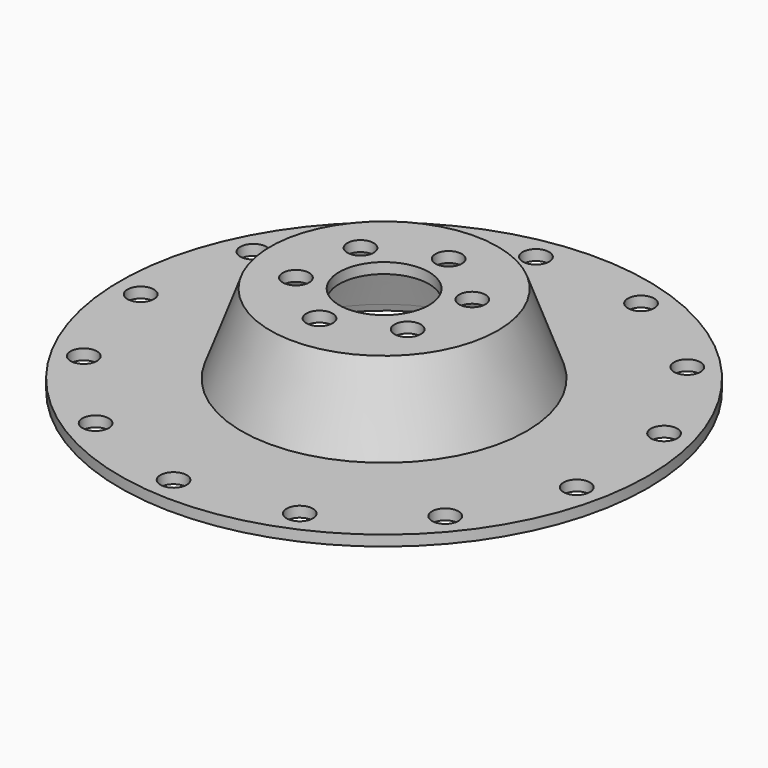
from build123d import *

# Parameters (mm, degrees)
F0_R      = 6.35
F1_DEPTH  = 0.254
F2_R      = 3.429
F3_DEPTH  = 1.905
F3_TAPER  = 20
F4_T      = 0.254
F5_R      = 1.0795
F6_DEPTH  = 25.4
F7_R      = 0.3175
F8_DEPTH  = 25.4
F9_R      = 0.3175
F10_DEPTH = 25.4


# Not quite as in the source:
# - a shell that OpenCascade refuses in one call is made with other operations: the cavity is built on its own and cut out


with BuildPart() as f1:
    # F0 (on Top) → F1 (new body)
    with BuildSketch(Plane.XY):
        Circle(F0_R)
    extrude(amount=F1_DEPTH)

    # F2 (on face) → F3 (join)
    with BuildSketch(Plane.XY.offset(0.254)):
        Circle(F2_R)
    extrude(amount=F3_DEPTH, taper=F3_TAPER)

    # F4: shell of thickness 0.254, made by hand


with BuildPart() as f4_core1:
    # F4_t2: copy of F1
    add(f1.part)

    # the walls: a layer under each face that stays
    f4_faces = [f4_core1.faces().sort_by_distance(p)[0] for p in [
        (-6.35, 0, 0.127),
        (-4.2333333333, -4.2333333333, 0.254),
        (-3.0823183519, 0, 1.2065),
        (0, 0, 2.159),
    ]]
    thicken(f4_faces, amount=-F4_T, mode=Mode.SUBTRACT)

    # F4_s3 → F4_t4 (revolve, cut)
    with BuildSketch(Plane.XZ):
        Polygon((3.4313868193, 0.2574087312), (3.429, 0), (3.2511472853, 0), (3.1903180743, 0.1671268836), align=None)
    revolve(axis=Axis((0, 0, 0.254), (0, 0, -1)), mode=Mode.SUBTRACT)


with BuildPart() as f1_1:
    add(f1.part)

    # what is left inside the walls is the cavity
    f4_cavity = [f4_core1.part.solids().sort_by_distance(p)[0] for p in [
        (-2.977087, 0, 0.745549),
    ]]
    add(f4_cavity, mode=Mode.SUBTRACT)

    # F5 (on face) → F6 (cut)
    with BuildSketch(Plane.XY.offset(2.159)):
        Circle(F5_R)
    extrude(amount=-F6_DEPTH, mode=Mode.SUBTRACT)

    # F7 (on face) → F8 (cut)
    with BuildSketch(Plane.XY.offset(2.159)):
        with Locations((-1.3804862777, 1.0167437666)):
            Circle(F7_R)
        with Locations((-1.5707690699, -0.6871643028)):
            Circle(F7_R)
        with Locations((-0.1902827922, -1.7039080694)):
            Circle(F7_R)
        with Locations((1.3804862777, -1.0167437666)):
            Circle(F7_R)
        with Locations((1.5707690699, 0.6871643028)):
            Circle(F7_R)
        with Locations((0.1902827922, 1.7039080694)):
            Circle(F7_R)
    extrude(amount=-F8_DEPTH, mode=Mode.SUBTRACT)

    # F9 (on face) → F10 (cut)
    with BuildSketch(Plane.XY.offset(0.254)):
        with Locations((-3.3923081987, 4.5992901719)):
            Circle(F9_R)
        with Locations((-5.1411364532, 2.4959849698)):
            Circle(F9_R)
        with Locations((-5.7121923037, -0.179120309)):
            Circle(F9_R)
        with Locations((-4.9746537368, -2.8131912837)):
            Circle(F9_R)
        with Locations((-3.0974819499, -4.8027940378)):
            Circle(F9_R)
        with Locations((-0.510714377, -5.6921345579)):
            Circle(F9_R)
        with Locations((2.193051705, -5.2774756484)):
            Circle(F9_R)
        with Locations((4.3944160704, -3.6538106683)):
            Circle(F9_R)
        with Locations((5.5890726726, -1.1931016973)):
            Circle(F9_R)
        with Locations((5.5033400811, 1.5409324941)):
            Circle(F9_R)
        with Locations((4.1568585995, 3.9219576214)):
            Circle(F9_R)
        with Locations((1.8580909083, 5.4045095223)):
            Circle(F9_R)
        with Locations((-0.8663430176, 5.6489534231)):
            Circle(F9_R)
    extrude(amount=-F10_DEPTH, mode=Mode.SUBTRACT)


solid = f1_1.part
